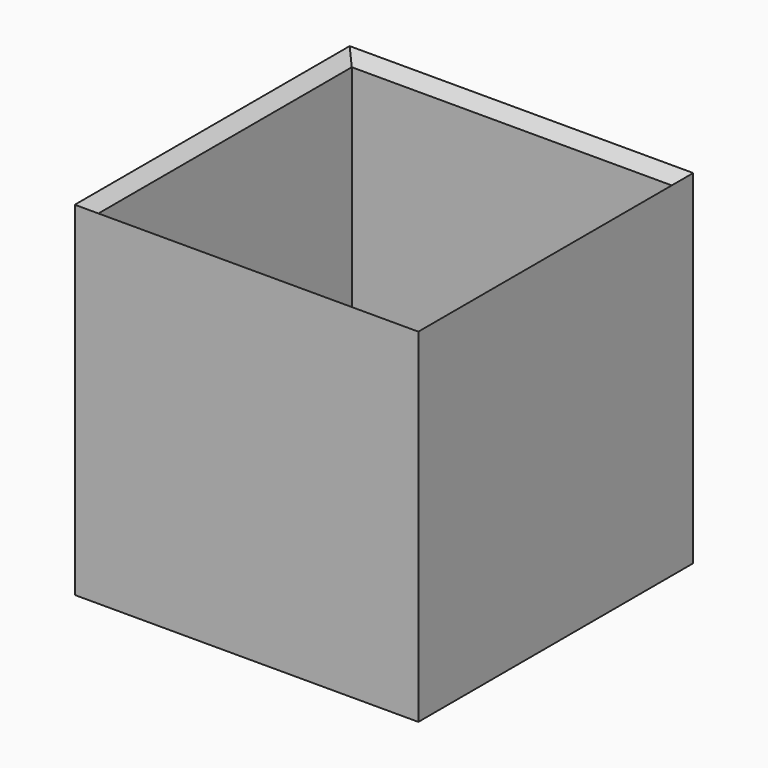
from build123d import *

# Parameters (mm, degrees)
F0_W         = 40.64
F0_H         = 40.64
F1_DEPTH     = 44.45
F2_T         = -1.27
F3_T1_DEPTH  = 38.1
F3_T3_DEPTH  = 38.1
F3_T9_DEPTH  = 51.1641495789
F3_T15_DEPTH = 51.1641495789
F3_T24_DEPTH = 51.1641495789
F3_T30_DEPTH = 51.1641495789
F3_T39_DEPTH = 51.1641495789
F3_T45_DEPTH = 51.1641495789
F3_T54_DEPTH = 51.1641495789
F3_T60_DEPTH = 51.1641495789


# Not quite as in the source:
# - a fillet or chamfer that OpenCascade refuses, or shapes differently, is made with other operations: its cross-section is extruded or revolved along the edge and cut away or added


with BuildPart() as f1:
    # F0 (on Top) → F1 (new body)
    with BuildSketch(Plane.XY):
        with Locations((-1.2905509211, 8.1801498235)):
            Rectangle(F0_W, F0_H)
    extrude(amount=F1_DEPTH)

    # F2
    f2_openings = [f1.faces().sort_by_distance(p)[0] for p in [
        (-1.290551, 8.18015, 44.45),
    ]]
    offset(amount=F2_T, openings=f2_openings)

    # F3: chamfer of 5.08 on 4 edges, made by hand

    # F3_s2 → F3_t1 (cut)
    with BuildSketch(Plane.XZ.offset(-27.2301498235)):
        Polygon((-25.4205509211, 44.45), (-20.3405509211, 39.37), (-20.3405509211, 44.45), align=None)
        Polygon((22.8394490789, 44.45), (17.7594490789, 39.37), (17.7594490789, 44.45), align=None)
    extrude(amount=F3_T1_DEPTH, mode=Mode.SUBTRACT)

    # F3_s4 → F3_t3 (cut)
    with BuildSketch(Plane.YZ.offset(-20.3405509211)):
        Polygon((32.3101498235, 44.45), (27.2301498235, 39.37), (27.2301498235, 44.45), align=None)
        Polygon((-15.9498501765, 44.45), (-10.8698501765, 39.37), (-10.8698501765, 44.45), align=None)
    extrude(amount=F3_T3_DEPTH, mode=Mode.SUBTRACT)


with BuildPart() as f3_tool7:
    # F3_s8 → F3_t9 (new body)
    with BuildSketch(Plane.YZ.offset(17.7594490789)):
        Polygon((32.3101498235, 44.45), (27.2301498235, 39.37), (27.2301498235, 44.45), align=None)
    extrude(amount=-F3_T9_DEPTH)

    split(bisect_by=Plane.XZ.offset(-28.5001498235), keep=Keep.TOP)

    split(bisect_by=Plane.YZ.offset(-21.6105509211), keep=Keep.TOP)

    split(bisect_by=Plane.YZ.offset(-20.3405509211), keep=Keep.BOTTOM)


with BuildPart() as f3_tool13:
    # F3_s14 → F3_t15 (new body)
    with BuildSketch(Plane.XZ.offset(-40.2942994024)):
        Polygon((-25.4205509211, 44.45), (-20.3405509211, 39.37), (-20.3405509211, 44.45), align=None)
    extrude(amount=F3_T15_DEPTH)

    split(bisect_by=Plane.XZ.offset(-28.5001498235), keep=Keep.TOP)

    split(bisect_by=Plane.YZ.offset(-21.6105509211), keep=Keep.TOP)

    split(bisect_by=Plane.XZ.offset(-27.2301498235), keep=Keep.BOTTOM)


with BuildPart() as f3_tool7_1:
    add(f3_tool7.part)

    # F3_t19: intersect F3_tool13
    add(f3_tool13.part, mode=Mode.INTERSECT)


with BuildPart() as f1_1:
    add(f1.part)

    # F3_t5: cut F3_tool7
    add(f3_tool7_1.part, mode=Mode.SUBTRACT)


with BuildPart() as f3_tool22:
    # F3_s23 → F3_t24 (new body)
    with BuildSketch(Plane.YZ.offset(-33.4047005)):
        Polygon((-15.9498501765, 44.45), (-10.8698501765, 39.37), (-10.8698501765, 44.45), align=None)
    extrude(amount=F3_T24_DEPTH)

    split(bisect_by=Plane.YZ.offset(-21.6105509211), keep=Keep.TOP)

    split(bisect_by=Plane.XZ.offset(12.1398501765), keep=Keep.BOTTOM)

    split(bisect_by=Plane.YZ.offset(-20.3405509211), keep=Keep.BOTTOM)


with BuildPart() as f3_tool28:
    # F3_s29 → F3_t30 (new body)
    with BuildSketch(Plane.XZ.offset(-27.2301498235)):
        Polygon((-25.4205509211, 44.45), (-20.3405509211, 39.37), (-20.3405509211, 44.45), align=None)
    extrude(amount=F3_T30_DEPTH)

    split(bisect_by=Plane.YZ.offset(-21.6105509211), keep=Keep.TOP)

    split(bisect_by=Plane.XZ.offset(12.1398501765), keep=Keep.BOTTOM)

    split(bisect_by=Plane.XZ.offset(10.8698501765), keep=Keep.TOP)


with BuildPart() as f3_tool22_1:
    add(f3_tool22.part)

    # F3_t34: intersect F3_tool28
    add(f3_tool28.part, mode=Mode.INTERSECT)


with BuildPart() as f1_2:
    add(f1_1.part)

    # F3_t20: cut F3_tool22
    add(f3_tool22_1.part, mode=Mode.SUBTRACT)


with BuildPart() as f3_tool37:
    # F3_s38 → F3_t39 (new body)
    with BuildSketch(Plane.YZ.offset(30.8235986578)):
        Polygon((32.3101498235, 44.45), (27.2301498235, 39.37), (27.2301498235, 44.45), align=None)
    extrude(amount=-F3_T39_DEPTH)

    split(bisect_by=Plane.XZ.offset(-28.5001498235), keep=Keep.TOP)

    split(bisect_by=Plane.YZ.offset(19.0294490789), keep=Keep.BOTTOM)

    split(bisect_by=Plane.YZ.offset(17.7594490789), keep=Keep.TOP)


with BuildPart() as f3_tool43:
    # F3_s44 → F3_t45 (new body)
    with BuildSketch(Plane.XZ.offset(10.8698501765)):
        Polygon((22.8394490789, 44.45), (17.7594490789, 39.37), (17.7594490789, 44.45), align=None)
    extrude(amount=-F3_T45_DEPTH)

    split(bisect_by=Plane.XZ.offset(-28.5001498235), keep=Keep.TOP)

    split(bisect_by=Plane.YZ.offset(19.0294490789), keep=Keep.BOTTOM)

    split(bisect_by=Plane.XZ.offset(-27.2301498235), keep=Keep.BOTTOM)


with BuildPart() as f3_tool37_1:
    add(f3_tool37.part)

    # F3_t49: intersect F3_tool43
    add(f3_tool43.part, mode=Mode.INTERSECT)


with BuildPart() as f1_3:
    add(f1_2.part)

    # F3_t35: cut F3_tool37
    add(f3_tool37_1.part, mode=Mode.SUBTRACT)


with BuildPart() as f3_tool52:
    # F3_s53 → F3_t54 (new body)
    with BuildSketch(Plane.XZ.offset(23.9339997554)):
        Polygon((22.8394490789, 44.45), (17.7594490789, 39.37), (17.7594490789, 44.45), align=None)
    extrude(amount=-F3_T54_DEPTH)

    split(bisect_by=Plane.XZ.offset(12.1398501765), keep=Keep.BOTTOM)

    split(bisect_by=Plane.YZ.offset(19.0294490789), keep=Keep.BOTTOM)

    split(bisect_by=Plane.XZ.offset(10.8698501765), keep=Keep.TOP)


with BuildPart() as f3_tool58:
    # F3_s59 → F3_t60 (new body)
    with BuildSketch(Plane.YZ.offset(-20.3405509211)):
        Polygon((-15.9498501765, 44.45), (-10.8698501765, 39.37), (-10.8698501765, 44.45), align=None)
    extrude(amount=F3_T60_DEPTH)

    split(bisect_by=Plane.XZ.offset(12.1398501765), keep=Keep.BOTTOM)

    split(bisect_by=Plane.YZ.offset(19.0294490789), keep=Keep.BOTTOM)

    split(bisect_by=Plane.YZ.offset(17.7594490789), keep=Keep.TOP)


with BuildPart() as f3_tool52_1:
    add(f3_tool52.part)

    # F3_t64: intersect F3_tool58
    add(f3_tool58.part, mode=Mode.INTERSECT)


with BuildPart() as f1_4:
    add(f1_3.part)

    # F3_t50: cut F3_tool52
    add(f3_tool52_1.part, mode=Mode.SUBTRACT)


solid = f1_4.part
